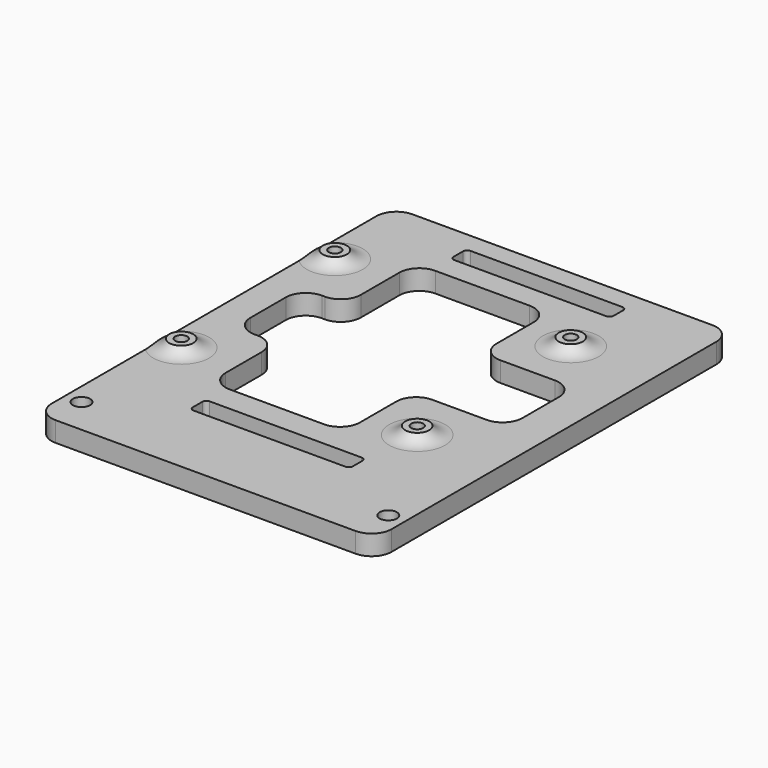
from build123d import *

# Parameters (mm, degrees)
F0_R     = 2.15
F0_R_2   = 3
F0_R_3   = 1.5
F0_R_4   = 5
F1_DEPTH = 5
F2_R     = 1
F3_R     = 5
F4_DEPTH = 7
F6_W     = 10.780302342
F6_H     = 21.0312269628
F6_W_2   = 23.6080475152
F6_H_2   = 21.3501416147
F7_DEPTH = 25
F8_R     = 5


# Not quite as in the source:
# - a fillet or chamfer that OpenCascade refuses, or shapes differently, is made with other operations: its cross-section is extruded or revolved along the edge and cut away or added


with BuildPart() as f1:
    # F0 (on Top) → F1 (new body)
    with BuildSketch(Plane.XY):
        Polygon((-29.2560231508, 20), (-29.2560231508, 0), (55.7439768492, 0), (55.7439768492, 20), (33.2439768492, 20), (-6.7560231508, 20), align=None)
        with Locations((-25.1060231508, 9.15)):
            Circle(F0_R, mode=Mode.SUBTRACT)
        with Locations((51.5939768492, 9.15)):
            Circle(F0_R, mode=Mode.SUBTRACT)
        Polygon((-29.2560231508, 106.5), (-29.2560231508, 20), (-6.7560231508, 20), (-6.7560231508, 25), (33.2439768492, 25), (33.2439768492, 20), (55.7439768492, 20), (55.7439768492, 106.5), (33.2439768492, 106.5), (33.2439768492, 101.5), (-6.7560231508, 101.5), (-6.7560231508, 106.5), align=None)
        with Locations((-24.2560231508, 39.25)):
            Circle(F0_R_2, mode=Mode.SUBTRACT)
        with Locations((3.2439768492, 53.25)):
            Circle(F0_R_3, mode=Mode.SUBTRACT)
        with Locations((23.2439768492, 53.25)):
            Circle(F0_R_3, mode=Mode.SUBTRACT)
        with Locations((34.7439768492, 39.25)):
            Circle(F0_R_2, mode=Mode.SUBTRACT)
        with Locations((13.2439768492, 63.25)):
            Circle(F0_R_4, mode=Mode.SUBTRACT)
        with Locations((3.2439768492, 73.25)):
            Circle(F0_R_3, mode=Mode.SUBTRACT)
        with Locations((-24.2560231508, 87.25)):
            Circle(F0_R_2, mode=Mode.SUBTRACT)
        with Locations((23.2439768492, 73.25)):
            Circle(F0_R_3, mode=Mode.SUBTRACT)
        with Locations((34.7439768492, 87.25)):
            Circle(F0_R_2, mode=Mode.SUBTRACT)
        Polygon((-29.2560231508, 111.5), (-29.2560231508, 106.5), (-6.7560231508, 106.5), (33.2439768492, 106.5), (55.7439768492, 106.5), (55.7439768492, 111.5), align=None)
        with Locations((-24.2560231508, 39.25)):
            Circle(F0_R_2)
        with Locations((-24.2560231508, 39.25)):
            Circle(F0_R_3, mode=Mode.SUBTRACT)
        with Locations((-24.2560231508, 87.25)):
            Circle(F0_R_2)
        with Locations((-24.2560231508, 87.25)):
            Circle(F0_R_3, mode=Mode.SUBTRACT)
        with Locations((34.7439768492, 39.25)):
            Circle(F0_R_2)
        with Locations((34.7439768492, 39.25)):
            Circle(F0_R_3, mode=Mode.SUBTRACT)
        with Locations((34.7439768492, 87.25)):
            Circle(F0_R_2)
        with Locations((34.7439768492, 87.25)):
            Circle(F0_R_3, mode=Mode.SUBTRACT)
        with Locations((13.2439768492, 63.25)):
            Circle(F0_R_4)
        with Locations((3.2439768492, 73.25)):
            Circle(F0_R_3)
        with Locations((3.2439768492, 53.25)):
            Circle(F0_R_3)
        with Locations((23.2439768492, 53.25)):
            Circle(F0_R_3)
        with Locations((23.2439768492, 73.25)):
            Circle(F0_R_3)
    extrude(amount=F1_DEPTH)

    # F2
    f2_edges = [f1.edges().sort_by_distance(p)[0] for p in [
        (-6.756023, 25, 2.5),
        (33.243977, 25, 2.5),
        (-6.756023, 20, 2.5),
        (33.243977, 20, 2.5),
        (-6.756023, 101.5, 2.5),
        (-6.756023, 106.5, 2.5),
        (33.243977, 106.5, 2.5),
        (33.243977, 101.5, 2.5),
    ]]
    fillet(f2_edges, radius=F2_R)

    # F3
    f3_edges = [f1.edges().sort_by_distance(p)[0] for p in [
        (-29.256023, 0, 2.5),
        (55.743977, 0, 2.5),
        (55.743977, 111.5, 2.5),
        (-29.256023, 111.5, 2.5),
    ]]
    fillet(f3_edges, radius=F3_R)

    # F0 (on Top) → F4 (join)
    with BuildSketch(Plane.XY):
        with Locations((-24.2560231508, 87.25)):
            Circle(F0_R_2)
        with Locations((-24.2560231508, 87.25)):
            Circle(F0_R_3, mode=Mode.SUBTRACT)
        with Locations((-24.2560231508, 39.25)):
            Circle(F0_R_2)
        with Locations((-24.2560231508, 39.25)):
            Circle(F0_R_3, mode=Mode.SUBTRACT)
        with Locations((34.7439768492, 87.25)):
            Circle(F0_R_2)
        with Locations((34.7439768492, 87.25)):
            Circle(F0_R_3, mode=Mode.SUBTRACT)
        with Locations((34.7439768492, 39.25)):
            Circle(F0_R_2)
        with Locations((34.7439768492, 39.25)):
            Circle(F0_R_3, mode=Mode.SUBTRACT)
    extrude(amount=F4_DEPTH)

    # F5: fillet of radius 5 on 4 edges, made by hand


with BuildPart() as f5_tool2:
    # F5_s3 → F5_t4 (revolve)
    with BuildSketch(Plane.XZ.offset(-87.25)):
        with BuildLine():
            ThreePointArc((-17.2560231508, 5), (-19.4920911283, 5.527864045), (-21.2560231508, 7))
            Line((-21.2560231508, 7), (-21.3360231508, 6.94))
            ThreePointArc((-21.3360231508, 6.94), (-21.3560231508, 6), (-21.3560231508, 5))
            Line((-21.3560231508, 5), (-21.2560231508, 4.9))
            Line((-21.2560231508, 4.9), (-17.2560231508, 4.9))
            Line((-17.2560231508, 4.9), (-17.2560231508, 5))
        make_face()
    revolve(axis=Axis((-24.2560231508, 87.25, 5), (0, 0, -1)))

    split(bisect_by=Plane.YZ.offset(-29.2560231508), keep=Keep.TOP)


with BuildPart() as f1_1:
    add(f1.part)

    # F5_t1: union F5_tool2
    add(f5_tool2.part)


with BuildPart() as f5_tool7:
    # F5_s8 → F5_t9 (revolve)
    with BuildSketch(Plane.XZ.offset(-39.25)):
        with BuildLine():
            ThreePointArc((-17.2560231508, 5), (-19.4920911283, 5.527864045), (-21.2560231508, 7))
            Line((-21.2560231508, 7), (-21.3360231508, 6.94))
            ThreePointArc((-21.3360231508, 6.94), (-21.3560231508, 6), (-21.3560231508, 5))
            Line((-21.3560231508, 5), (-21.2560231508, 4.9))
            Line((-21.2560231508, 4.9), (-17.2560231508, 4.9))
            Line((-17.2560231508, 4.9), (-17.2560231508, 5))
        make_face()
    revolve(axis=Axis((-24.2560231508, 39.25, 5), (0, 0, -1)))

    split(bisect_by=Plane.YZ.offset(-29.2560231508), keep=Keep.TOP)


with BuildPart() as f1_2:
    add(f1_1.part)

    # F5_t6: union F5_tool7
    add(f5_tool7.part)

    # F5_s11 → F5_t12 (revolve)
    with BuildSketch(Plane.XZ.offset(-39.25)):
        with BuildLine():
            ThreePointArc((41.7439768492, 5), (39.5079088717, 5.527864045), (37.7439768492, 7))
            Line((37.7439768492, 7), (37.6639768492, 6.94))
            ThreePointArc((37.6639768492, 6.94), (37.6439768492, 6), (37.6439768492, 5))
            Line((37.6439768492, 5), (37.7439768492, 4.9))
            Line((37.7439768492, 4.9), (41.7439768492, 4.9))
            Line((41.7439768492, 4.9), (41.7439768492, 5))
        make_face()
    revolve(axis=Axis((34.7439768492, 39.25, 5), (0, 0, -1)))

    # F5_s13 → F5_t14 (revolve)
    with BuildSketch(Plane.XZ.offset(-87.25)):
        with BuildLine():
            ThreePointArc((37.7439768492, 7), (39.5079088717, 5.527864045), (41.7439768492, 5))
            Line((41.7439768492, 5), (41.7439768492, 4.9))
            Line((41.7439768492, 4.9), (37.7439768492, 4.9))
            Line((37.7439768492, 4.9), (37.6439768492, 5))
            ThreePointArc((37.6439768492, 5), (37.6439768492, 6), (37.6639768492, 6.94))
            Line((37.6639768492, 6.94), (37.7439768492, 7))
        make_face()
    revolve(axis=Axis((34.7439768492, 87.25, 5), (0, 0, -1)))

    # F6 (on face) → F7 (cut)
    with BuildSketch(Plane.XY.offset(5)):
        Polygon((22.7412616368, 95.6321507692), (-10.8403607737, 95.6321507692), (-10.8403607737, 73.6251212656), (-10.8403607737, 52.5938943028), (-10.8403607737, 31.3930846751), (22.7412616368, 31.3930846751), (22.7412616368, 52.6874549687), (22.7412616368, 74.0375965834), align=None)
        with Locations((-16.2305119447, 63.1095077842)):
            Rectangle(F6_W, F6_H)
        with Locations((34.5452853944, 63.362525776)):
            Rectangle(F6_W_2, F6_H_2)
    extrude(amount=-F7_DEPTH, mode=Mode.SUBTRACT)

    # F8
    f8_edges = [f1_2.edges().sort_by_distance(p)[0] for p in [
        (-10.840361, 73.625121, 2.5),
        (22.741262, 74.037597, 2.5),
        (22.741262, 52.687455, 2.5),
        (-10.840361, 52.593894, 2.5),
        (-21.620663, 52.593894, 2.5),
        (-21.620663, 73.625121, 2.5),
        (-10.840361, 95.632151, 2.5),
        (22.741262, 95.632151, 2.5),
        (46.349309, 74.037597, 2.5),
        (46.349309, 52.687455, 2.5),
        (22.741262, 31.393085, 2.5),
        (-10.840361, 31.393085, 2.5),
    ]]
    fillet(f8_edges, radius=F8_R)


solid = f1_2.part
